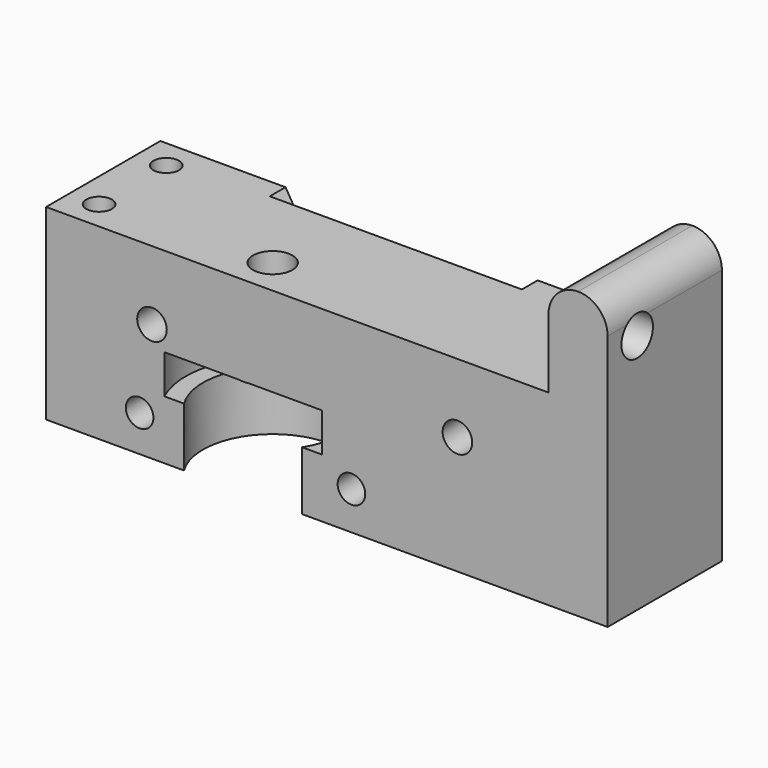
from build123d import *

# Parameters (mm, degrees)
F0_W         = 47
F0_H         = 14.5
F0_R         = 1.3
F0_R_2       = 2
F1_DEPTH     = 19
F4_DEPTH     = 9.9
F5_R         = 1.5
F5_R_2       = 1.4
F6_DEPTH     = 14.5
F7_DEPTH     = 10
F8_W         = 6
F8_H         = 14.5
F9_DEPTH     = 10
F10_R        = 2
F11_DEPTH    = 6
F12_T1_DEPTH = 29.5
F14_DEPTH    = 2


# Not quite as in the source:
# - a fillet or chamfer that OpenCascade refuses, or shapes differently, is made with other operations: its cross-section is extruded or revolved along the edge and cut away or added


with BuildPart() as f1:
    # F0 (on Top) → F1 (new body)
    with BuildSketch(Plane.XY):
        with Locations((3.5, 3.5)):
            Rectangle(F0_W, F0_H)
        with Locations((-17.01, -0.76)):
            Circle(F0_R, mode=Mode.SUBTRACT)
        Circle(F0_R_2, mode=Mode.SUBTRACT)
        with Locations((-17.01, 7.76)):
            Circle(F0_R, mode=Mode.SUBTRACT)
    extrude(amount=F1_DEPTH)

    # F2 (on face) → F3 (revolve, cut)
    with BuildSketch(Plane.XZ.offset(3.75)):
        Polygon((0, 9.93), (-7.995, 9.93), (-7.995, 5.98), (-5.995, 5.98), (-5.995, 0), (0, 0), align=None)
    revolve(axis=Axis((0, 0, 0), (0, 0, 1)), mode=Mode.SUBTRACT)

    # F4 (cut): a face of the model
    f4_faces = [f1.faces().sort_by_distance(p)[0] for p in [
        (0, 3.6439339828, 0),
    ]]
    extrude(f4_faces, amount=-F4_DEPTH, mode=Mode.SUBTRACT)

    # F5 (on face) → F6 (cut, through all)
    with BuildSketch(Plane.XZ.offset(3.75)):
        with Locations((-9.25, 12)):
            Circle(F5_R)
        with Locations((-10.5055273842, 3.7)):
            Circle(F5_R_2)
        with Locations((10.9938158954, 3.8680432901)):
            Circle(F5_R_2)
        with Locations((21.75, 12)):
            Circle(F5_R)
    extrude(amount=-F6_DEPTH, mode=Mode.SUBTRACT)

    # F7 (add): a face of the model
    f7_faces = [f1.faces().sort_by_distance(p)[0] for p in [
        (27, 3.5, 9.5),
    ]]
    extrude(f7_faces, amount=F7_DEPTH)

    # F8 (on face) → F9 (join)
    with BuildSketch(Plane.XY.offset(19)):
        with Locations((34, 3.5)):
            Rectangle(F8_W, F8_H)
    extrude(amount=F9_DEPTH)

    # F10 (on face) → F11 (cut, through all)
    with BuildSketch(Plane.YZ.offset(37)):
        with Locations((0, 24.5)):
            Circle(F10_R)
    extrude(amount=-F11_DEPTH, mode=Mode.SUBTRACT)

    # F12: fillet of radius 3 on 2 edges, made by hand

    # F12_s2 → F12_t1 (cut)
    with BuildSketch(Plane.XZ.offset(-18.25)):
        with BuildLine():
            ThreePointArc((31, 26), (31.8786796564, 28.1213203436), (34, 29))
            Line((34, 29), (31, 29))
            Line((31, 29), (31, 26))
        make_face()
        with BuildLine():
            ThreePointArc((34, 29), (36.1213203436, 28.1213203436), (37, 26))
            Line((37, 26), (37, 29))
            Line((37, 29), (34, 29))
        make_face()
    extrude(amount=F12_T1_DEPTH, mode=Mode.SUBTRACT)

    # F13 (on face) → F14 (cut)
    with BuildSketch(Plane(origin=(0, 10.75, 0), x_dir=(-1, 0, 0), z_dir=(0, 1, 0))):
        with BuildLine():
            Line((7.2936857888, 19), (-18.2936857888, 19))
            ThreePointArc((-18.2936857888, 19), (-5.5, 11.3063278591), (7.2936857888, 19))
        make_face()
    extrude(amount=-F14_DEPTH, mode=Mode.SUBTRACT)


solid = f1.part
